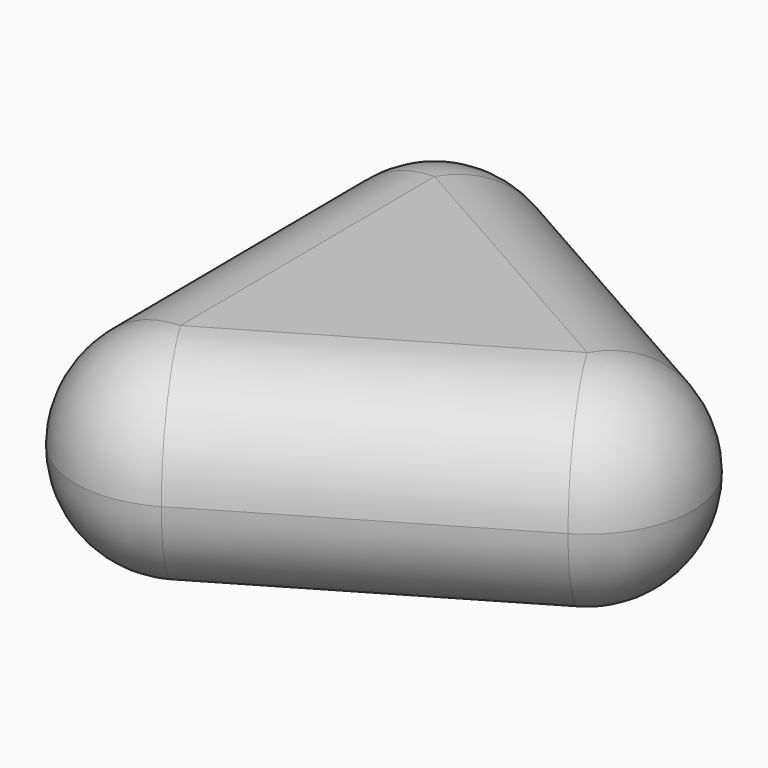
from build123d import *

# Parameters (mm, degrees)
F1_DEPTH = 10.16
F2_R     = 5.08
F3_R     = 5.07999


# Not quite as in the source:
# - a fillet or chamfer is up to 0.001 mm smaller than in the source, because OpenCascade refuses the exact size


with BuildPart() as f1:
    # F0 (on Top) → F1 (new body)
    with BuildSketch(Plane.XY):
        Polygon((19.1086118392, 0.1538227311), (-9.6875203124, 16.4716319182), (-9.4210915267, -16.6254546493), align=None)
    extrude(amount=F1_DEPTH)

    # F2
    f2_edges = [f1.edges().sort_by_distance(p)[0] for p in [
        (-9.421092, -16.625455, 5.08),
        (19.108612, 0.153823, 5.08),
        (-9.68752, 16.471632, 5.08),
    ]]
    fillet(f2_edges, radius=F2_R)

    # F3 (radius 5.08 in the source; OpenCascade refuses exactly that, so slightly less here)
    f3_edges = [f1.edges().sort_by_distance(p)[0] for p in [
        (4.84376, -8.235816, 0),
        (-6.916588, -12.205742, 0),
        (14.028776, 0.11293, 0),
        (-9.554306, -0.076911, 0),
        (4.710546, 8.312727, 0),
        (-7.112189, 12.092812, 0),
        (4.84376, -8.235816, 10.16),
        (-6.916588, -12.205742, 10.16),
        (14.028776, 0.11293, 10.16),
        (-9.554306, -0.076911, 10.16),
        (4.710546, 8.312727, 10.16),
        (-7.112189, 12.092812, 10.16),
    ]]
    fillet(f3_edges, radius=F3_R)


solid = f1.part
